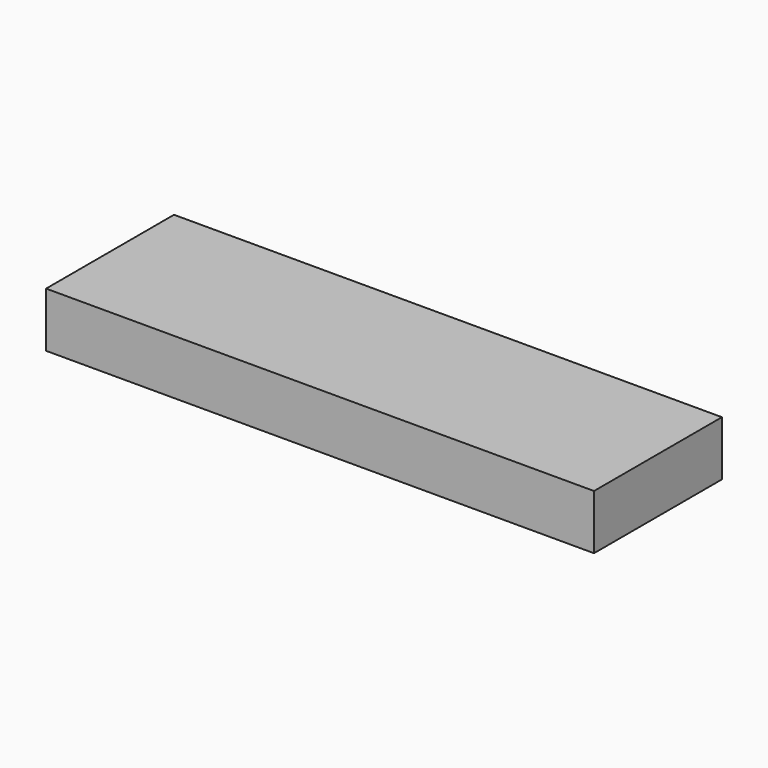
from build123d import *

# Parameters (mm, degrees)
F0_W         = 25.4
F0_H         = 7.4115503722
F0_W_2       = 0.4408832231
F0_H_2       = 3.7935884112
F1_DEPTH     = 2.032
F0_TEXT_SIZE = 5.3138467568
F2_DEPTH     = 2.54


# Not quite as in the source:
# - Text() gives the source's letters only with a copy of the font that has no kerning and outlines rounded to 1/6400 em; it was checked with that copy


with BuildPart() as f1:
    # F0 (on Top) → F1 (new body)
    with BuildSketch(Plane.XY):
        with Locations((-11.78155342, 1.8302188876)):
            Rectangle(F0_W, F0_H)
        with BuildLine():
            Line((-21.4455231065, 1.3542006344), (-20.5787018543, 3.7935884112))
            Line((-20.5787018543, 3.7935884112), (-20.104607089, 3.7935884112))
            Line((-20.104607089, 3.7935884112), (-21.4712620518, 0))
            Line((-21.4712620518, 0), (-21.9071635435, 0))
            Line((-21.9071635435, 0), (-23.2671761979, 3.7935884112))
            Line((-23.2671761979, 3.7935884112), (-22.799723741, 3.7935884112))
            Line((-22.799723741, 3.7935884112), (-21.9279207574, 1.3392554404))
            add(Edge.make_bspline(
                [(-21.9279207574, 1.3392554404), (-21.7776385288, 0.915808277), (-21.6896279419, 0.5164394817)],
                knots=[0, 0, 0, 1, 1, 1], degree=2))
            add(Edge.make_bspline(
                [(-21.6896279419, 0.5164394817), (-21.5958053351, 0.9365654909), (-21.4455231065, 1.3542006344)],
                knots=[0, 0, 0, 1, 1, 1], degree=2))
        make_face(mode=Mode.SUBTRACT)
        Polygon((-16.7419384382, 0), (-17.1985971439, 0), (-17.6710313321, 1.2064092715), (-19.1912896777, 1.2064092715), (-19.657911846, 0), (-20.104607089, 0), (-18.6051059573, 3.8093638938), (-18.2339669729, 3.8093638938), align=None, mode=Mode.SUBTRACT)
        Polygon((-14.1057722737, 0), (-16.2205172252, 0), (-16.2205172252, 3.7935884112), (-15.7796340021, 3.7935884112), (-15.7796340021, 0.3993687953), (-14.1057722737, 0.3993687953), align=None, mode=Mode.SUBTRACT)
        Polygon((-12.3048763963, 2.1454656281), (-10.722346409, 0), (-11.2412767563, 0), (-12.6237072017, 1.8399194395), (-13.0214154199, 1.4870468034), (-13.0214154199, 0), (-13.462298643, 0), (-13.462298643, 3.7935884112), (-13.0214154199, 3.7935884112), (-13.0214154199, 1.9121545439), (-11.3010575324, 3.7935884112), (-10.7796363193, 3.7935884112), align=None, mode=Mode.SUBTRACT)
        Polygon((-10.2399487581, 3.7935884112), (-9.2352996056, 1.8963790613), (-8.2240081447, 3.7935884112), (-7.7465922252, 3.7935884112), (-9.0127822727, 1.4712713208), (-9.0127822727, 0), (-9.4586472271, 0), (-9.4586472271, 1.4505141069), (-10.722346409, 3.7935884112), align=None, mode=Mode.SUBTRACT)
        with BuildLine():
            Line((-5.9921925069, 1.5775482559), (-6.7842877891, 1.5775482559))
            Line((-6.7842877891, 1.5775482559), (-6.7842877891, 0))
            Line((-6.7842877891, 0), (-7.2251710122, 0))
            Line((-7.2251710122, 0), (-7.2251710122, 3.7935884112))
            Line((-7.2251710122, 3.7935884112), (-6.1848194518, 3.7935884112))
            add(Edge.make_bspline(
                [(-6.1848194518, 3.7935884112), (-5.4865467764, 3.7935884112), (-5.1531859213, 3.5262354963)],
                knots=[0, 0, 0, 1, 1, 1], degree=2))
            add(Edge.make_bspline(
                [(-5.1531859213, 3.5262354963), (-4.8198250661, 3.2588825813), (-4.8198250661, 2.7216858858)],
                knots=[0, 0, 0, 1, 1, 1], degree=2))
            add(Edge.make_bspline(
                [(-4.8198250661, 2.7216858858), (-4.8198250661, 1.9694444542), (-5.5828602489, 1.704582405)],
                knots=[0, 0, 0, 1, 1, 1], degree=2))
            Line((-5.5828602489, 1.704582405), (-4.5524721512, 0))
            Line((-4.5524721512, 0), (-5.0738933642, 0))
            Line((-5.0738933642, 0), (-5.9921925069, 1.5775482559))
        make_face(mode=Mode.SUBTRACT)
        with Locations((-3.7201078741, 1.8967942056)):
            Rectangle(F0_W_2, F0_H_2, mode=Mode.SUBTRACT)
        Polygon((-0.3445697506, 0.394387064), (-0.3445697506, 0), (-2.4593147021, 0), (-2.4593147021, 3.7935884112), (-0.3445697506, 3.7935884112), (-0.3445697506, 3.4016922129), (-2.018431479, 3.4016922129), (-2.018431479, 2.1795074589), (-0.4458649544, 2.1795074589), (-0.4458649544, 1.7901021262), (-2.018431479, 1.7901021262), (-2.018431479, 0.394387064), align=None, mode=Mode.SUBTRACT)
    extrude(amount=F1_DEPTH)


with BuildPart() as f2:
    # F0 (on Top) → F2 (new body)
    with BuildSketch(Plane.XY):
        with Locations((-11.78155342, 1.8302188876)):
            Rectangle(F0_W, F0_H)
        with BuildLine():
            Line((-21.4455231065, 1.3542006344), (-20.5787018543, 3.7935884112))
            Line((-20.5787018543, 3.7935884112), (-20.104607089, 3.7935884112))
            Line((-20.104607089, 3.7935884112), (-21.4712620518, 0))
            Line((-21.4712620518, 0), (-21.9071635435, 0))
            Line((-21.9071635435, 0), (-23.2671761979, 3.7935884112))
            Line((-23.2671761979, 3.7935884112), (-22.799723741, 3.7935884112))
            Line((-22.799723741, 3.7935884112), (-21.9279207574, 1.3392554404))
            add(Edge.make_bspline(
                [(-21.9279207574, 1.3392554404), (-21.7776385288, 0.915808277), (-21.6896279419, 0.5164394817)],
                knots=[0, 0, 0, 1, 1, 1], degree=2))
            add(Edge.make_bspline(
                [(-21.6896279419, 0.5164394817), (-21.5958053351, 0.9365654909), (-21.4455231065, 1.3542006344)],
                knots=[0, 0, 0, 1, 1, 1], degree=2))
        make_face(mode=Mode.SUBTRACT)
        Polygon((-16.7419384382, 0), (-17.1985971439, 0), (-17.6710313321, 1.2064092715), (-19.1912896777, 1.2064092715), (-19.657911846, 0), (-20.104607089, 0), (-18.6051059573, 3.8093638938), (-18.2339669729, 3.8093638938), align=None, mode=Mode.SUBTRACT)
        Polygon((-14.1057722737, 0), (-16.2205172252, 0), (-16.2205172252, 3.7935884112), (-15.7796340021, 3.7935884112), (-15.7796340021, 0.3993687953), (-14.1057722737, 0.3993687953), align=None, mode=Mode.SUBTRACT)
        Polygon((-12.3048763963, 2.1454656281), (-10.722346409, 0), (-11.2412767563, 0), (-12.6237072017, 1.8399194395), (-13.0214154199, 1.4870468034), (-13.0214154199, 0), (-13.462298643, 0), (-13.462298643, 3.7935884112), (-13.0214154199, 3.7935884112), (-13.0214154199, 1.9121545439), (-11.3010575324, 3.7935884112), (-10.7796363193, 3.7935884112), align=None, mode=Mode.SUBTRACT)
        Polygon((-10.2399487581, 3.7935884112), (-9.2352996056, 1.8963790613), (-8.2240081447, 3.7935884112), (-7.7465922252, 3.7935884112), (-9.0127822727, 1.4712713208), (-9.0127822727, 0), (-9.4586472271, 0), (-9.4586472271, 1.4505141069), (-10.722346409, 3.7935884112), align=None, mode=Mode.SUBTRACT)
        with BuildLine():
            Line((-5.9921925069, 1.5775482559), (-6.7842877891, 1.5775482559))
            Line((-6.7842877891, 1.5775482559), (-6.7842877891, 0))
            Line((-6.7842877891, 0), (-7.2251710122, 0))
            Line((-7.2251710122, 0), (-7.2251710122, 3.7935884112))
            Line((-7.2251710122, 3.7935884112), (-6.1848194518, 3.7935884112))
            add(Edge.make_bspline(
                [(-6.1848194518, 3.7935884112), (-5.4865467764, 3.7935884112), (-5.1531859213, 3.5262354963)],
                knots=[0, 0, 0, 1, 1, 1], degree=2))
            add(Edge.make_bspline(
                [(-5.1531859213, 3.5262354963), (-4.8198250661, 3.2588825813), (-4.8198250661, 2.7216858858)],
                knots=[0, 0, 0, 1, 1, 1], degree=2))
            add(Edge.make_bspline(
                [(-4.8198250661, 2.7216858858), (-4.8198250661, 1.9694444542), (-5.5828602489, 1.704582405)],
                knots=[0, 0, 0, 1, 1, 1], degree=2))
            Line((-5.5828602489, 1.704582405), (-4.5524721512, 0))
            Line((-4.5524721512, 0), (-5.0738933642, 0))
            Line((-5.0738933642, 0), (-5.9921925069, 1.5775482559))
        make_face(mode=Mode.SUBTRACT)
        with Locations((-3.7201078741, 1.8967942056)):
            Rectangle(F0_W_2, F0_H_2, mode=Mode.SUBTRACT)
        Polygon((-0.3445697506, 0.394387064), (-0.3445697506, 0), (-2.4593147021, 0), (-2.4593147021, 3.7935884112), (-0.3445697506, 3.7935884112), (-0.3445697506, 3.4016922129), (-2.018431479, 3.4016922129), (-2.018431479, 2.1795074589), (-0.4458649544, 2.1795074589), (-0.4458649544, 1.7901021262), (-2.018431479, 1.7901021262), (-2.018431479, 0.394387064), align=None, mode=Mode.SUBTRACT)
        with BuildLine():
            Line((-6.7842877891, 3.4066739443), (-6.7842877891, 1.9561598374))
            Line((-6.7842877891, 1.9561598374), (-6.1790074319, 1.9561598374))
            add(Edge.make_bspline(
                [(-6.1790074319, 1.9561598374), (-5.7123852636, 1.9561598374), (-5.4944345177, 2.1417293296)],
                knots=[0, 0, 0, 1, 1, 1], degree=2))
            add(Edge.make_bspline(
                [(-5.4944345177, 2.1417293296), (-5.2764837718, 2.3272988218), (-5.2764837718, 2.6984378062)],
                knots=[0, 0, 0, 1, 1, 1], degree=2))
            add(Edge.make_bspline(
                [(-5.2764837718, 2.6984378062), (-5.2764837718, 3.074558522), (-5.4981708162, 3.2406162331)],
                knots=[0, 0, 0, 1, 1, 1], degree=2))
            add(Edge.make_bspline(
                [(-5.4981708162, 3.2406162331), (-5.7198578606, 3.4066739443), (-6.210558397, 3.4066739443)],
                knots=[0, 0, 0, 1, 1, 1], degree=2))
            Line((-6.210558397, 3.4066739443), (-6.7842877891, 3.4066739443))
        make_face()
        with Locations((-23.2671761979, 0)):
            Text('VALKYRIE', F0_TEXT_SIZE, font='Open Sans', text_align=(TextAlign.LEFT, TextAlign.BOTTOM))
        with BuildLine():
            Line((-19.0351954292, 1.6032872012), (-17.8080289438, 1.6032872012))
            Line((-17.8080289438, 1.6032872012), (-18.2497424554, 2.7789757961))
            add(Edge.make_bspline(
                [(-18.2497424554, 2.7789757961), (-18.3352621767, 3.0023234176), (-18.4257636293, 3.3261359543)],
                knots=[0, 0, 0, 1, 1, 1], degree=2))
            add(Edge.make_bspline(
                [(-18.4257636293, 3.3261359543), (-18.4830535396, 3.0770493876), (-18.5893304748, 2.7789757961)],
                knots=[0, 0, 0, 1, 1, 1], degree=2))
            Line((-18.5893304748, 2.7789757961), (-19.0351954292, 1.6032872012))
        make_face()
    extrude(amount=F2_DEPTH)


solid = Compound([f1.part, f2.part])
